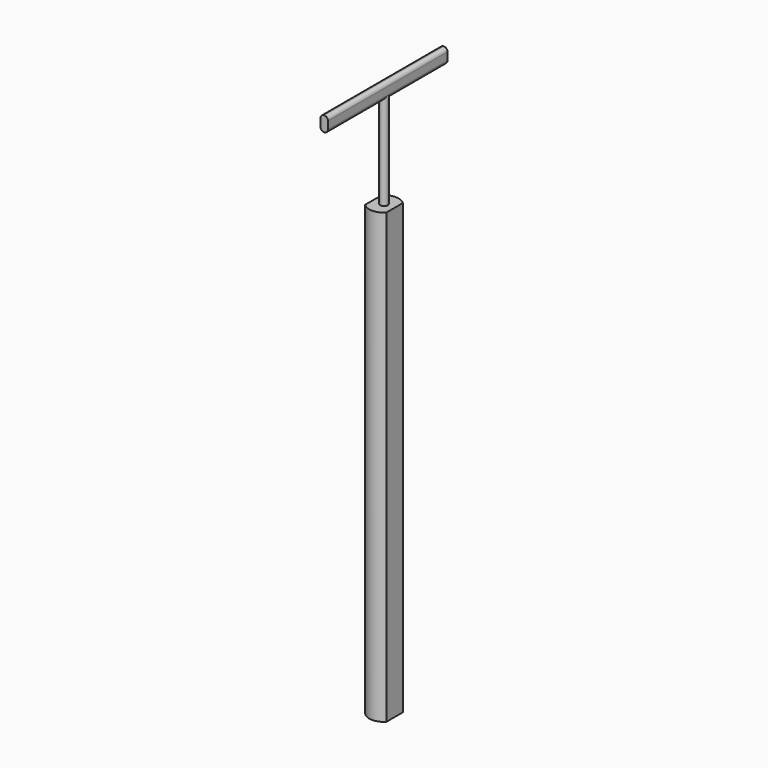
from build123d import *

# Parameters (mm, degrees)
F0_R         = 3.95
F1_DEPTH     = 120
F3_DEPTH     = 120.001
F4_R         = 1
F5_DEPTH     = 25
F6_W         = 2
F6_H         = 40
F7_DEPTH     = 4
F8_T1_DEPTH  = 45
F8_T6_DEPTH  = 22.5
F8_S7_R      = 1
F8_T8_DEPTH  = 13
F8_T12_DEPTH = 22.5
F8_S13_R     = 1
F8_T14_DEPTH = 13
F8_T18_DEPTH = 22.5
F8_S19_R     = 1
F8_T20_DEPTH = 13
F8_T24_DEPTH = 22.5
F8_S25_R     = 1
F8_T26_DEPTH = 13


# Not quite as in the source:
# - a fillet or chamfer that OpenCascade refuses, or shapes differently, is made with other operations: its cross-section is extruded or revolved along the edge and cut away or added


with BuildPart() as f1:
    # F0 (on Top) → F1 (new body)
    with BuildSketch(Plane.XY):
        Circle(F0_R)
    extrude(amount=F1_DEPTH)

    # F2 (on face) → F3 (cut, through all)
    with BuildSketch(Plane.XY.offset(120)):
        with BuildLine():
            Line((-2.8354893758, -2.75), (-2.8354893758, 2.75))
            ThreePointArc((-2.8354893758, 2.75), (-3.95, 0), (-2.8354893758, -2.75))
        make_face()
        with BuildLine():
            ThreePointArc((3.95, 0), (3.6607842762, 1.4836301705), (2.8354893758, 2.75))
            Line((2.8354893758, 2.75), (2.8354893758, -2.75))
            ThreePointArc((2.8354893758, -2.75), (3.6607842762, -1.4836301705), (3.95, 0))
        make_face()
    extrude(amount=-F3_DEPTH, mode=Mode.SUBTRACT)

    # F4 (on face) → F5 (join)
    with BuildSketch(Plane.XY.offset(120)):
        Circle(F4_R)
    extrude(amount=F5_DEPTH)

    # F6 (on face) → F7 (join)
    with BuildSketch(Plane.XY.offset(145)):
        Rectangle(F6_W, F6_H)
    extrude(amount=F7_DEPTH)

    # F8: fillet of radius 1 on 6 edges, made by hand

    # F8_s2 → F8_t1 (cut)
    with BuildSketch(Plane.XZ.offset(-22.5)):
        with BuildLine():
            ThreePointArc((1, 148), (0.7071067812, 148.7071067812), (0, 149))
            Line((0, 149), (1, 149))
            Line((1, 149), (1, 148))
        make_face()
        with BuildLine():
            ThreePointArc((-1, 148), (-0.7071067812, 148.7071067812), (0, 149))
            Line((0, 149), (-1, 149))
            Line((-1, 149), (-1, 148))
        make_face()
    extrude(amount=F8_T1_DEPTH, mode=Mode.SUBTRACT)


with BuildPart() as f8_tool4:
    # F8_s5 → F8_t6 (new body)
    with BuildSketch(Plane.XZ.offset(22.5)):
        with BuildLine():
            ThreePointArc((0, 145), (0.7071067812, 145.2928932188), (1, 146))
            Line((1, 146), (1, 145))
            Line((1, 145), (0, 145))
        make_face()
    extrude(amount=-F8_T6_DEPTH)

    # F8_s7 → F8_t8 (cut, symmetric)
    with BuildSketch(Plane.XY.offset(145.5)):
        Circle(F8_S7_R)
    extrude(amount=F8_T8_DEPTH, both=True, mode=Mode.SUBTRACT)


with BuildPart() as f1_1:
    add(f1.part)

    # F8_t3: cut F8_tool4
    add(f8_tool4.part, mode=Mode.SUBTRACT)


with BuildPart() as f8_tool10:
    # F8_s11 → F8_t12 (new body)
    with BuildSketch(Plane.XZ):
        with BuildLine():
            ThreePointArc((0, 145), (-0.7071067812, 145.2928932188), (-1, 146))
            Line((-1, 146), (-1, 145))
            Line((-1, 145), (0, 145))
        make_face()
    extrude(amount=F8_T12_DEPTH)

    # F8_s13 → F8_t14 (cut, symmetric)
    with BuildSketch(Plane.XY.offset(145.5)):
        Circle(F8_S13_R)
    extrude(amount=F8_T14_DEPTH, both=True, mode=Mode.SUBTRACT)


with BuildPart() as f1_2:
    add(f1_1.part)

    # F8_t9: cut F8_tool10
    add(f8_tool10.part, mode=Mode.SUBTRACT)


with BuildPart() as f8_tool16:
    # F8_s17 → F8_t18 (new body)
    with BuildSketch(Plane.XZ.offset(-22.5)):
        with BuildLine():
            ThreePointArc((0, 145), (-0.7071067812, 145.2928932188), (-1, 146))
            Line((-1, 146), (-1, 145))
            Line((-1, 145), (0, 145))
        make_face()
    extrude(amount=F8_T18_DEPTH)

    # F8_s19 → F8_t20 (cut, symmetric)
    with BuildSketch(Plane.XY.offset(145.5)):
        Circle(F8_S19_R)
    extrude(amount=F8_T20_DEPTH, both=True, mode=Mode.SUBTRACT)


with BuildPart() as f1_3:
    add(f1_2.part)

    # F8_t15: cut F8_tool16
    add(f8_tool16.part, mode=Mode.SUBTRACT)


with BuildPart() as f8_tool22:
    # F8_s23 → F8_t24 (new body)
    with BuildSketch(Plane.XZ):
        with BuildLine():
            ThreePointArc((0, 145), (0.7071067812, 145.2928932188), (1, 146))
            Line((1, 146), (1, 145))
            Line((1, 145), (0, 145))
        make_face()
    extrude(amount=-F8_T24_DEPTH)

    # F8_s25 → F8_t26 (cut, symmetric)
    with BuildSketch(Plane.XY.offset(145.5)):
        Circle(F8_S25_R)
    extrude(amount=F8_T26_DEPTH, both=True, mode=Mode.SUBTRACT)


with BuildPart() as f1_4:
    add(f1_3.part)

    # F8_t21: cut F8_tool22
    add(f8_tool22.part, mode=Mode.SUBTRACT)


solid = f1_4.part
